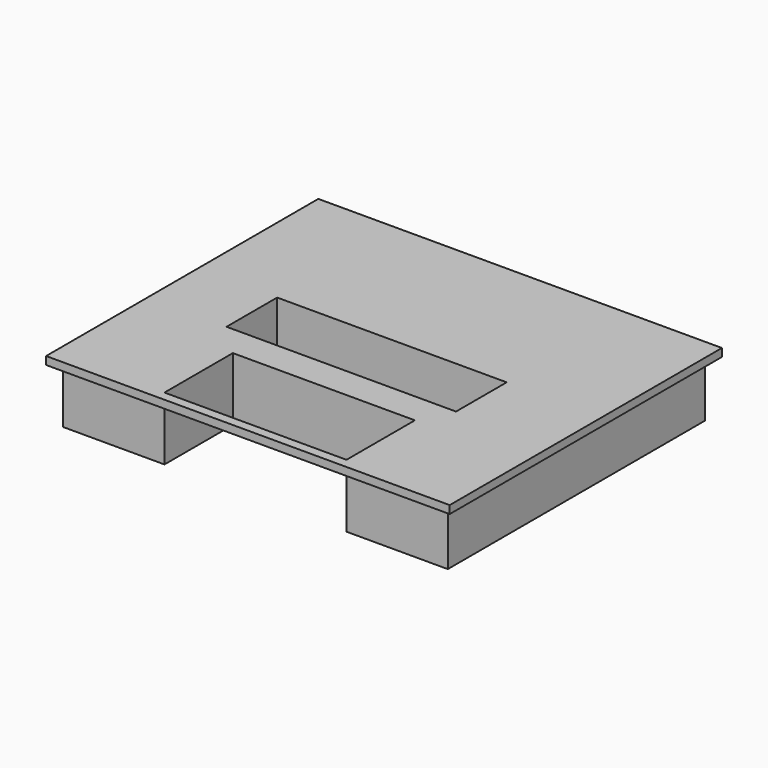
from build123d import *

# Parameters (mm, degrees)
F0_W     = 51
F0_H     = 43
F1_DEPTH = 1
F2_W     = 31
F2_H     = 10
F2_W_2   = 29
F2_H_2   = 8
F3_DEPTH = 7
F4_DEPTH = 25
F2_W_3   = 23
F2_H_3   = 1
F2_H_4   = 9.8
F5_DEPTH = 25


with BuildPart() as f1:
    # F0 (on Top) → F1 (new body)
    with BuildSketch(Plane.XY):
        Rectangle(F0_W, F0_H)
    extrude(amount=F1_DEPTH)

    # F2 (on face) → F3 (join)
    with BuildSketch(Plane(origin=(0, 0, 0), x_dir=(1, 0, 0), z_dir=(0, 0, -1))):
        Polygon((-11.5, 19.3), (-11.5, 20.3), (-24.3, 20.3), (-24.3, 14.5), (-23.3, 14.5), (-23.3, 19.3), (-12.5, 19.3), align=None)
        Polygon((19.5, -20.3), (24.3, -20.3), (24.3, 20.3), (11.5, 20.3), (11.5, 19.3), (12.5, 19.3), (23.3, 19.3), (23.3, -19.3), (19.5, -19.3), align=None)
        Polygon((-24.3, -20.3), (-19.5, -20.3), (-19.5, -19.3), (-23.3, -19.3), (-23.3, 1.5), (-24.3, 1.5), align=None)
        with Locations((-1, 1.5)):
            Rectangle(F2_W, F2_H)
        with Locations((-1, 1.5)):
            Rectangle(F2_W_2, F2_H_2, mode=Mode.SUBTRACT)
        Polygon((12.5, 19.3), (11.5, 19.3), (11.5, 9.5), (-11.5, 9.5), (-11.5, 19.3), (-12.5, 19.3), (-12.5, 8.5), (12.5, 8.5), align=None)
    extrude(amount=F3_DEPTH)

    # F4 (cut): a face of the model
    f4_faces = [f1.faces().sort_by_distance(p)[0] for p in [
        (-1, -1.5, 0),
    ]]
    extrude(f4_faces, amount=-F4_DEPTH, mode=Mode.SUBTRACT)

    # F2 (on face) → F5 (cut)
    with BuildSketch(Plane(origin=(0, 0, 0), x_dir=(1, 0, 0), z_dir=(0, 0, -1))):
        with Locations((0, 19.8)):
            Rectangle(F2_W_3, F2_H_3)
        with Locations((0, 14.4)):
            Rectangle(F2_W_3, F2_H_4)
    extrude(amount=-F5_DEPTH, mode=Mode.SUBTRACT)


solid = f1.part
